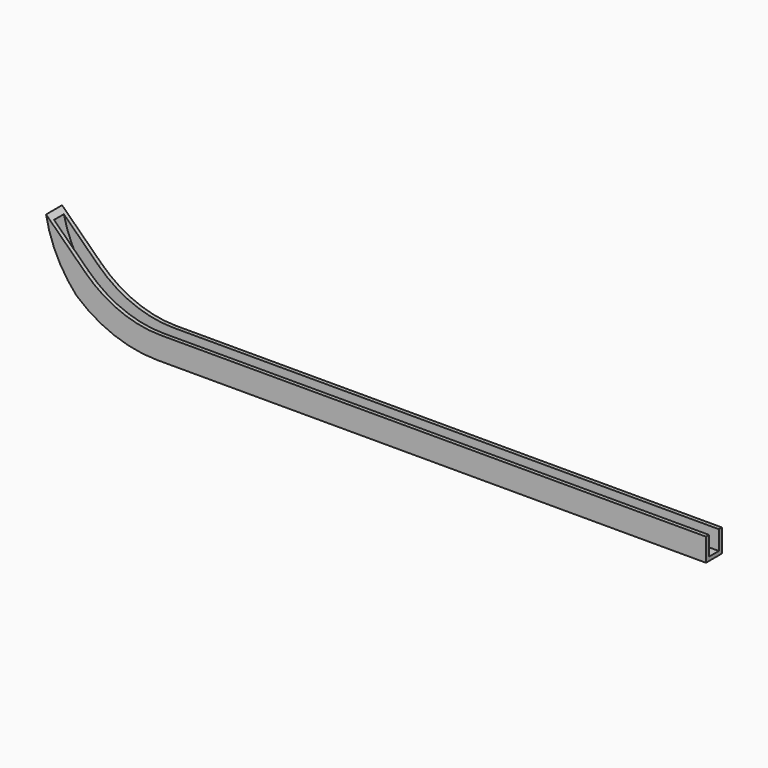
from build123d import *

# Parameters (mm, degrees)
F3_DEPTH    = 6.5
F4_T1_DEPTH = 87.9231463955
F4_T3_DEPTH = 86.4923799402
F5_R        = 35
F6_T        = -1.25


# Not quite as in the source:
# - a fillet or chamfer that OpenCascade refuses, or shapes differently, is made with other operations: its cross-section is extruded or revolved along the edge and cut away or added


with BuildPart() as f3:
    # F2 (on Front) → F3 (new body)
    with BuildSketch(Plane.XZ):
        Polygon((0, 19.5199243858), (20, 0), (215, 0), (215, 7.5), (23.0533679898, 7.5), (0, 30), align=None)
    extrude(amount=F3_DEPTH)

    # F4: fillet of radius 40 on 2 edges, made by hand

    # F4_s2 → F4_t1 (cut)
    with BuildSketch(Plane.XZ.offset(-40.7115731978)):
        with BuildLine():
            ThreePointArc((8.3460077876, 11.374252339), (21.2020218527, 2.9525310821), (36.2846292791, 0))
            Line((36.2846292791, 0), (20, 0))
            Line((20, 0), (8.3460077876, 11.374252339))
        make_face()
    extrude(amount=F4_T1_DEPTH, mode=Mode.SUBTRACT)

    # F4_s4 → F4_t3 (cut)
    with BuildSketch(Plane.XZ.offset(-39.9961899701)):
        with BuildLine():
            ThreePointArc((11.4492084149, 8.345540259), (4.0262452257, 18.2748088699), (0, 30))
            Line((0, 30), (0, 19.5199243858))
            Line((0, 19.5199243858), (11.4492084149, 8.345540259))
        make_face()
    extrude(amount=F4_T3_DEPTH, mode=Mode.SUBTRACT)

    # F5
    f5_edges = [f3.edges().sort_by_distance(p)[0] for p in [
        (23.053368, -3.25, 7.5),
    ]]
    fillet(f5_edges, radius=F5_R)

    # F6
    f6_openings = [f3.faces().sort_by_distance(p)[0] for p in [
        (6.428062, -3.25, 23.726235),
        (24.105137, -3.25, 10.083465),
        (126.151209, -3.25, 7.5),
        (215, -3.25, 3.75),
    ]]
    offset(amount=F6_T, openings=f6_openings)


solid = f3.part
